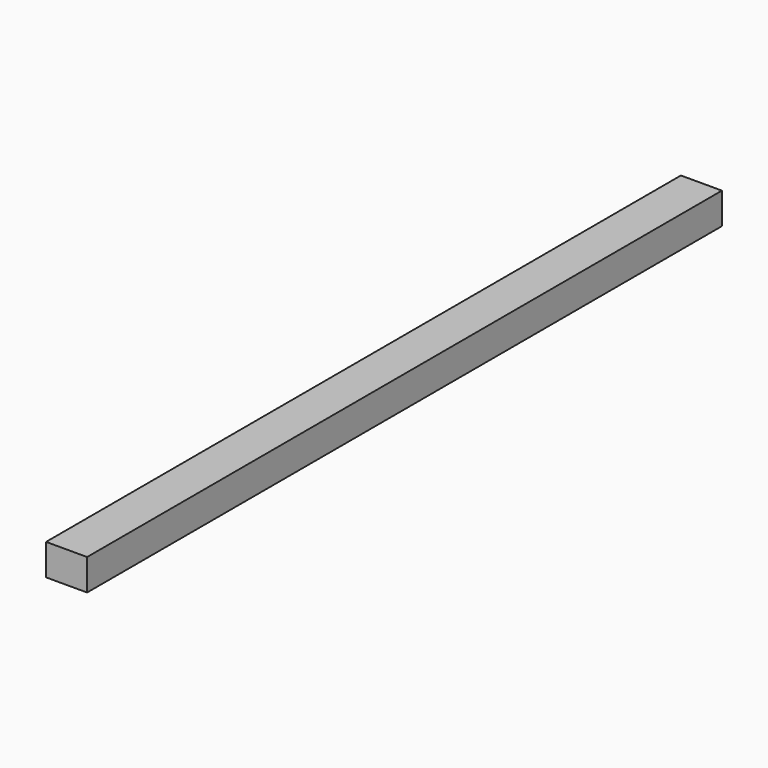
from build123d import *

# Parameters (mm, degrees)
F2_W     = 16.6624
F2_H     = 12.7
F3_DEPTH = 322.2752


# Not quite as in the source:
# - a variable given as a bare number and used for a length is read in inches; the dataset says mm whatever the document's units were


with BuildPart() as f3:
    # F2 (on Front) → F3 (new body)
    with BuildSketch(Plane.XZ):
        with Locations((8.3312, -6.35)):
            Rectangle(F2_W, F2_H)
    extrude(amount=F3_DEPTH)


solid = f3.part
